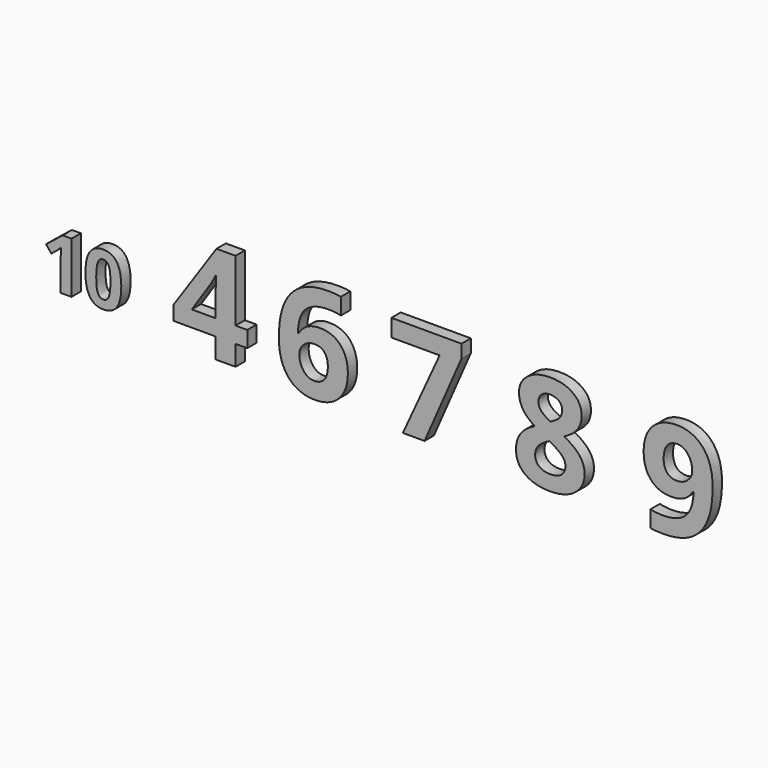
from build123d import *

# Parameters (mm, degrees)
F0_TEXT_SIZE  = 74.4517038889
F1_DEPTH      = 6.35
F2_TEXT_SIZE  = 74.4517038889
F3_DEPTH      = 6.35
F4_TEXT_SIZE  = 74.4517038889
F5_DEPTH      = 6.35
F6_TEXT_SIZE  = 74.4517038889
F7_DEPTH      = 6.35
F8_TEXT_SIZE  = 74.4517038889
F9_DEPTH      = 6.35
F10_TEXT_SIZE = 39.0508474576
F11_DEPTH     = 6.35


# Not quite as in the source:
# - Text() gives the source's letters only with a copy of the font that has no kerning and outlines rounded to 1/6400 em; it was checked with that copy


with BuildPart() as f1:
    # F0 (on Front) → F1 (new body)
    with BuildSketch(Plane.XZ):
        with Locations((-117.6725825045, -32.5941771348)):
            Text('4', F0_TEXT_SIZE, font='Open Sans', font_style=FontStyle.BOLD, text_align=(TextAlign.LEFT, TextAlign.BOTTOM))
    extrude(amount=F1_DEPTH)


with BuildPart() as f3:
    # F2 (on Front) → F3 (new body)
    with BuildSketch(Plane.XZ):
        with Locations((-61.8154184902, -33.6362429424)):
            Text('6', F2_TEXT_SIZE, font='Open Sans', font_style=FontStyle.BOLD, text_align=(TextAlign.LEFT, TextAlign.BOTTOM))
    extrude(amount=F3_DEPTH)


with BuildPart() as f5:
    # F4 (on Front) → F5 (new body)
    with BuildSketch(Plane.XZ):
        with Locations((0, -34.6449962706)):
            Text('7', F4_TEXT_SIZE, font='Open Sans', font_style=FontStyle.BOLD, text_align=(TextAlign.LEFT, TextAlign.BOTTOM))
    extrude(amount=F5_DEPTH)


with BuildPart() as f7:
    # F6 (on Front) → F7 (new body)
    with BuildSketch(Plane.XZ):
        with Locations((67.1361360303, -35.8343476307)):
            Text('8', F6_TEXT_SIZE, font='Open Sans', font_style=FontStyle.BOLD, text_align=(TextAlign.LEFT, TextAlign.BOTTOM))
    extrude(amount=F7_DEPTH)


with BuildPart() as f9:
    # F8 (on Front) → F9 (new body)
    with BuildSketch(Plane.XZ):
        with Locations((136.7536840496, -36.1879346792)):
            Text('9', F8_TEXT_SIZE, font='Open Sans', font_style=FontStyle.BOLD, text_align=(TextAlign.LEFT, TextAlign.BOTTOM))
    extrude(amount=F9_DEPTH)


with BuildPart() as f11:
    # F10 (on Front) → F11 (new body)
    with BuildSketch(Plane.XZ):
        with Locations((-188.0256438518, -28.1166101695)):
            Text('10', F10_TEXT_SIZE, font='Open Sans', font_style=FontStyle.BOLD, text_align=(TextAlign.LEFT, TextAlign.BOTTOM))
    extrude(amount=F11_DEPTH)


solid = Compound([f1.part, f3.part, f5.part, f7.part, f9.part, f11.part])
